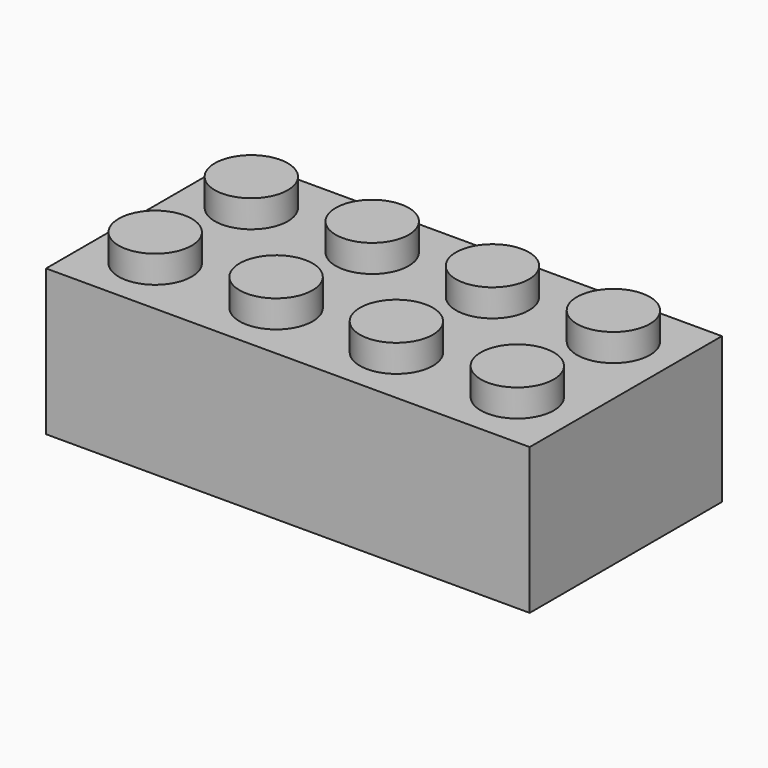
from build123d import *

# Parameters (mm, degrees)
F0_W     = 31.8
F0_H     = 9.6
F1_DEPTH = 15.8
F2_R     = 2.4
F3_DEPTH = 1.8
F4_W     = 29.4
F4_H     = 13.4
F4_R     = 3.25685
F5_DEPTH = 6.4


# Not quite as in the source:
# - the program builds the solid bodies; features that only make, move or delete a surface that nothing else refers to are left out


with BuildPart() as f1:
    # F0 (on Front) → F1 (new body)
    with BuildSketch(Plane.XZ):
        with Locations((7.8699710073, -4.8)):
            Rectangle(F0_W, F0_H)
    extrude(amount=F1_DEPTH)

    # F4 (on face) → F5 (cut)
    with BuildSketch(Plane(origin=(0, 0, -9.6), x_dir=(1, 0, 0), z_dir=(0, 0, -1))):
        with Locations((7.8699710073, 7.9)):
            Rectangle(F4_W, F4_H)
        with Locations((0, 7.9)):
            Circle(F4_R, mode=Mode.SUBTRACT)
        with Locations((7.8699710073, 7.9)):
            Circle(F4_R, mode=Mode.SUBTRACT)
        with Locations((15.8199710073, 7.9)):
            Circle(F4_R, mode=Mode.SUBTRACT)
    extrude(amount=-F5_DEPTH, mode=Mode.SUBTRACT)


with BuildPart() as f3:
    # F2 (on face) → F3 (new body)
    with BuildSketch(Plane.XY):
        with Locations((19.7949710073, -3.95)):
            Circle(F2_R)
    extrude(amount=F3_DEPTH)


with BuildPart() as f3b:
    # F2 (on face) → F3, piece 2 (new body)
    with BuildSketch(Plane.XY):
        with Locations((19.7949710073, -11.85)):
            Circle(F2_R)
    extrude(amount=F3_DEPTH)


with BuildPart() as f3c:
    # F2 (on face) → F3, piece 3 (new body)
    with BuildSketch(Plane.XY):
        with Locations((11.8449710073, -11.85)):
            Circle(F2_R)
    extrude(amount=F3_DEPTH)


with BuildPart() as f3d:
    # F2 (on face) → F3, piece 4 (new body)
    with BuildSketch(Plane.XY):
        with Locations((3.9349855036, -3.95)):
            Circle(F2_R)
    extrude(amount=F3_DEPTH)


with BuildPart() as f3e:
    # F2 (on face) → F3, piece 5 (new body)
    with BuildSketch(Plane.XY):
        with Locations((11.8449710073, -3.95)):
            Circle(F2_R)
    extrude(amount=F3_DEPTH)


with BuildPart() as f3f:
    # F2 (on face) → F3, piece 6 (new body)
    with BuildSketch(Plane.XY):
        with Locations((3.9349855036, -11.85)):
            Circle(F2_R)
    extrude(amount=F3_DEPTH)


with BuildPart() as f3g:
    # F2 (on face) → F3, piece 7 (new body)
    with BuildSketch(Plane.XY):
        with Locations((-4.0150144964, -11.85)):
            Circle(F2_R)
    extrude(amount=F3_DEPTH)


with BuildPart() as f3h:
    # F2 (on face) → F3, piece 8 (new body)
    with BuildSketch(Plane.XY):
        with Locations((-4.0150144964, -3.95)):
            Circle(F2_R)
    extrude(amount=F3_DEPTH)


solid = Compound([f1.part, f3.part, f3b.part, f3c.part, f3d.part, f3e.part, f3f.part, f3g.part, f3h.part])
